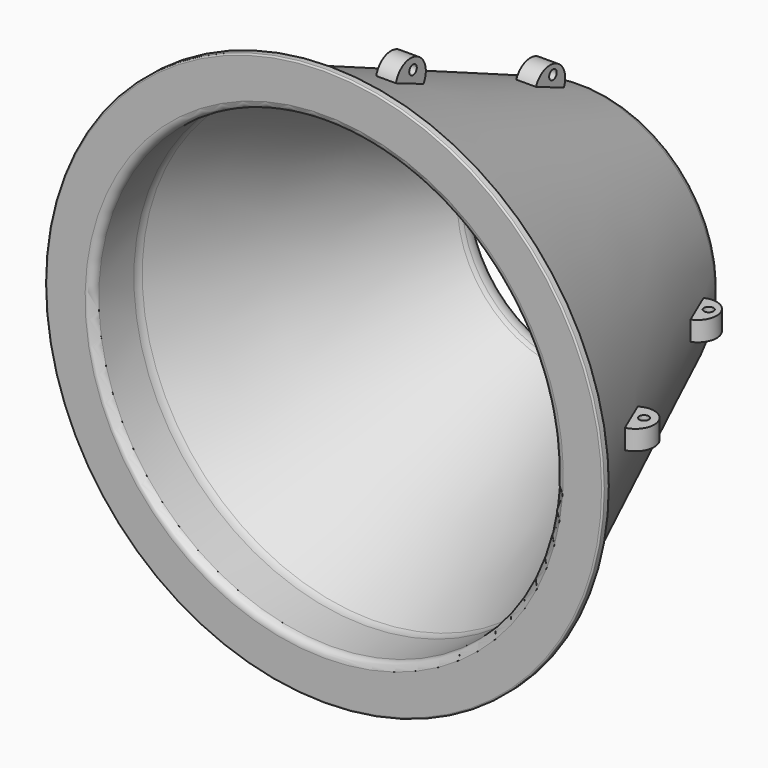
from build123d import *

# Parameters (mm, degrees)
F4_R      = 2.54
F5_R      = 0.5
F6_R      = 6.35
F7_DEPTH  = 3.302
F8_ANGLE  = -90
F9_DEPTH  = 3.302
F10_R     = 1.5884390158
F11_DEPTH = 12.7
F12_R     = 1.5875
F13_DEPTH = 12.7


# Not quite as in the source:
# - a fillet or chamfer that OpenCascade refuses, or shapes differently, is made with other operations: its cross-section is extruded or revolved along the edge and cut away or added


with BuildPart() as f2:
    # F1 (on Top) → F2 (revolve)
    with BuildSketch(Plane.XY):
        with BuildLine():
            Line((-93.5, 0), (-77.62, 0))
            Line((-77.62, 0), (-77.62, 17.2648650431))
            ThreePointArc((-77.62, 17.2648650431), (-77.4641828492, 18.6629347231), (-77.0043783212, 19.9923923608))
            Line((-77.0043783212, 19.9923923608), (-37.6156216788, 102.8036737445))
            ThreePointArc((-37.6156216788, 102.8036737445), (-37.1558171508, 104.1331313823), (-37, 105.5312010623))
            Line((-37, 105.5312010623), (-37, 110))
            Line((-37, 110), (-40.2242628687, 110))
            ThreePointArc((-40.2242628687, 110), (-43.7293858539, 108.9449610818), (-46.0697714652, 106.1304292467))
            Line((-46.0697714652, 106.1304292467), (-89.95, 2.72))
            Line((-89.95, 2.72), (-93.5, 2.72))
            Line((-93.5, 2.72), (-93.5, 0))
        make_face()
    revolve(axis=Axis((0, 28.3275991678, 0), (0, 1, 0)))

    # F3: fillet of radius 5.08 on 1 edges, made by hand

    # F3_s1 → F3_t2 (revolve, cut)
    with BuildSketch(Plane.XY):
        with BuildLine():
            ThreePointArc((-37.1245161297, 104.2798615477), (-37.6385377676, 107.7012594993), (-40.2242628687, 110))
            Line((-40.2242628687, 110), (-40.0361988329, 110.4719066841))
            ThreePointArc((-40.0361988329, 110.4719066841), (-38.6121314343, 110.508), (-37, 110.508))
            Line((-37, 110.508), (-36.492, 110))
            ThreePointArc((-36.492, 110), (-36.492, 105.5312010623), (-36.6264774201, 104.1797543865))
            Line((-36.6264774201, 104.1797543865), (-37.1245161297, 104.2798615477))
        make_face()
    revolve(axis=Axis((0, 110, 0), (0, 1, 0)), mode=Mode.SUBTRACT)

    # F4
    f4_edges = [f2.edges().sort_by_distance(p)[0] for p in [
        (77.62, 0, 0),
    ]]
    fillet(f4_edges, radius=F4_R)

    # F5
    f5_edges = [f2.edges().sort_by_distance(p)[0] for p in [
        (93.5, 2.72, 0),
        (93.5, 0, 0),
    ]]
    fillet(f5_edges, radius=F5_R)

    # F6 (on Top) → F7 (join, symmetric)
    with BuildSketch(Plane.XY):
        with Locations((-78.5837723943, 32.1033455817)):
            Circle(F6_R)
        with Locations((-52.7833043417, 90.5129020759)):
            Circle(F6_R)
        with Locations((52.7833043417, 90.5129020759)):
            Circle(F6_R)
        with Locations((78.5837723943, 32.1033455817)):
            Circle(F6_R)
    extrude(amount=F7_DEPTH, both=True)


with BuildPart() as f2_1:
    # F8: moved
    add(f2.part.rotate(Axis((0, 28.3275991678, 0), (0, 1, 0)), F8_ANGLE))

    # F6 (on Top) → F9 (join, symmetric)
    with BuildSketch(Plane.XY):
        with Locations((-78.5837723943, 32.1033455817)):
            Circle(F6_R)
        with Locations((-52.7833043417, 90.5129020759)):
            Circle(F6_R)
        with Locations((52.7833043417, 90.5129020759)):
            Circle(F6_R)
        with Locations((78.5837723943, 32.1033455817)):
            Circle(F6_R)
    extrude(amount=F9_DEPTH, both=True)

    # F10 (on face) → F11 (cut, symmetric)
    with BuildSketch(Plane(origin=(0, 0, -3.302), x_dir=(1, 0, 0), z_dir=(0, 0, -1))):
        with Locations((55.3165711462, -91.9873043895)):
            Circle(F10_R)
        with Locations((80.47170192, -33.4471799433)):
            Circle(F10_R)
        with Locations((-80.59284091, -32.9536646605)):
            Circle(F10_R)
        with Locations((-54.8363402486, -91.4571881294)):
            Circle(F10_R)
    extrude(amount=F11_DEPTH, both=True, mode=Mode.SUBTRACT)

    # F12 (on Right) → F13 (cut, symmetric)
    with BuildSketch(Plane.YZ):
        with Locations((33.0776236951, 81.0802206397)):
            Circle(F12_R)
        with Locations((91.7218402028, 55.8268986642)):
            Circle(F12_R)
        with Locations((91.6659608483, -55.79033494)):
            Circle(F12_R)
        with Locations((33.0493189394, -80.8606371284)):
            Circle(F12_R)
    extrude(amount=F13_DEPTH, both=True, mode=Mode.SUBTRACT)


solid = f2_1.part
